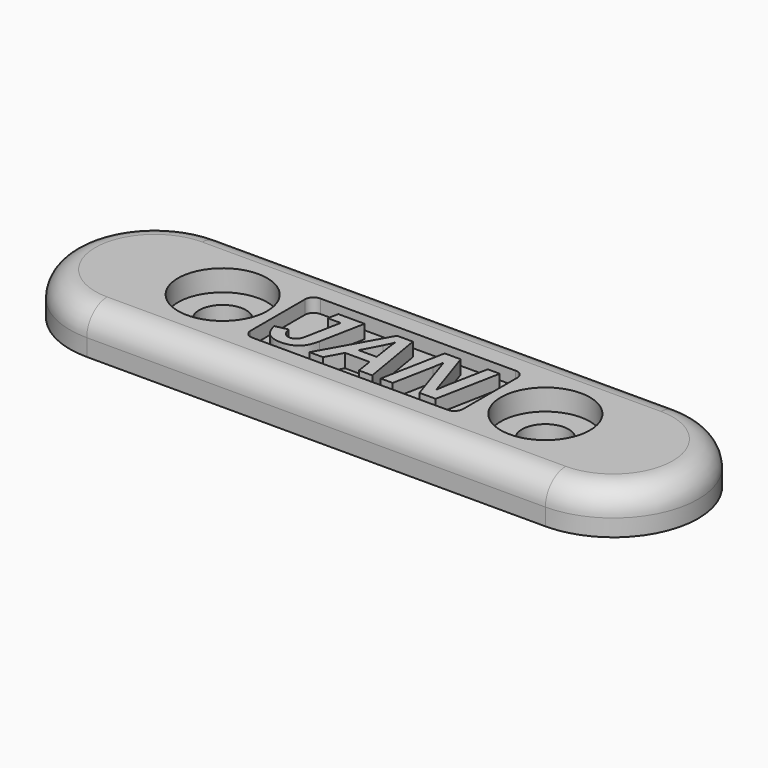
from build123d import *

# Parameters (mm, degrees)
F0_R     = 5.25
F0_R_2   = 2.75
F1_DEPTH = 5
F2_DEPTH = 2.5
F4_R     = 3
F6_DEPTH = 1.6


with BuildPart() as f1:
    # F0 (on Top) → F1 (new body)
    with BuildSketch(Plane.XY):
        with BuildLine():
            Line((27, 10), (-27, 10))
            ThreePointArc((-27, 10), (-37, 0), (-27, -10))
            Line((-27, -10), (27, -10))
            ThreePointArc((27, -10), (37, 0), (27, 10))
        make_face()
        with Locations((-19, 0)):
            Circle(F0_R, mode=Mode.SUBTRACT)
        with Locations((19, 0)):
            Circle(F0_R, mode=Mode.SUBTRACT)
        with Locations((-19, 0)):
            Circle(F0_R)
        with Locations((-19, 0)):
            Circle(F0_R_2, mode=Mode.SUBTRACT)
        with Locations((19, 0)):
            Circle(F0_R)
        with Locations((19, 0)):
            Circle(F0_R_2, mode=Mode.SUBTRACT)
    extrude(amount=-F1_DEPTH)

    # F0 (on Top) → F2 (cut)
    with BuildSketch(Plane.XY):
        with Locations((-19, 0)):
            Circle(F0_R)
        with Locations((-19, 0)):
            Circle(F0_R_2, mode=Mode.SUBTRACT)
        with Locations((19, 0)):
            Circle(F0_R)
        with Locations((19, 0)):
            Circle(F0_R_2, mode=Mode.SUBTRACT)
    extrude(amount=-F2_DEPTH, mode=Mode.SUBTRACT)

    # F4
    f4_edges = [f1.edges().sort_by_distance(p)[0] for p in [
        (0, -10, 0),
        (0, 10, 0),
    ]]
    fillet(f4_edges, radius=F4_R)

    # F5 (on face) → F6 (cut)
    with BuildSketch(Plane.XY):
        with BuildLine():
            Line((11.5, 5), (-11.5, 5))
            ThreePointArc((-11.5, 5), (-12.2071067812, 4.7071067812), (-12.5, 4))
            Line((-12.5, 4), (-12.5, -4))
            ThreePointArc((-12.5, -4), (-12.2071067812, -4.7071067812), (-11.5, -5))
            Line((-11.5, -5), (11.5, -5))
            ThreePointArc((11.5, -5), (12.2071067812, -4.7071067812), (12.5, -4))
            Line((12.5, -4), (12.5, 4))
            ThreePointArc((12.5, 4), (12.2071067812, 4.7071067812), (11.5, 5))
        make_face()
        with BuildLine():
            add(Edge.make_bspline(
                [(-7.1087151842, -3.5052785265), (-7.754492363, -4.0761455526), (-8.9168912848, -4.0761455526)],
                knots=[0, 0, 0, 1, 1, 1], degree=2))
            add(Edge.make_bspline(
                [(-8.9168912848, -4.0761455526), (-9.939802336, -4.0761455526), (-10.5502770291, -3.5586627733)],
                knots=[0, 0, 0, 1, 1, 1], degree=2))
            add(Edge.make_bspline(
                [(-10.5502770291, -3.5586627733), (-11.1607517221, -3.041179994), (-11.3656783468, -1.928721174)],
                knots=[0, 0, 0, 1, 1, 1], degree=2))
            Line((-11.3656783468, -1.928721174), (-9.9277478287, -1.6153039832))
            add(Edge.make_bspline(
                [(-9.9277478287, -1.6153039832), (-9.6814914645, -2.8328092243), (-8.8152890087, -2.8328092243)],
                knots=[0, 0, 0, 1, 1, 1], degree=2))
            add(Edge.make_bspline(
                [(-8.8152890087, -2.8328092243), (-8.5242587601, -2.8328092243), (-8.325359389, -2.7036537886)],
                knots=[0, 0, 0, 1, 1, 1], degree=2))
            add(Edge.make_bspline(
                [(-8.325359389, -2.7036537886), (-8.126460018, -2.5744983528), (-7.9973045822, -2.3377133872)],
                knots=[0, 0, 0, 1, 1, 1], degree=2))
            add(Edge.make_bspline(
                [(-7.9973045822, -2.3377133872), (-7.8681491465, -2.1009284217), (-7.7699910153, -1.5998053309)],
                knots=[0, 0, 0, 1, 1, 1], degree=2))
            Line((-7.7699910153, -1.5998053309), (-7.0002246181, 2.3712938005))
            Line((-7.0002246181, 2.3712938005), (-8.5139263252, 2.3712938005))
            Line((-8.5139263252, 2.3712938005), (-8.2762803235, 3.6146301288))
            Line((-8.2762803235, 3.6146301288), (-5.1817160827, 3.6146301288))
            Line((-5.1817160827, 3.6146301288), (-6.2201257862, -1.6910751722))
            add(Edge.make_bspline(
                [(-6.2201257862, -1.6910751722), (-6.4629380054, -2.9344115004), (-7.1087151842, -3.5052785265)],
                knots=[0, 0, 0, 1, 1, 1], degree=2))
        make_face(mode=Mode.SUBTRACT)
        Polygon((1.7909553759, -3.9676549865), (0.220425277, -3.9676549865), (-0.075771189, -2.0303234501), (-2.965408805, -2.0303234501), (-4.0141509434, -3.9676549865), (-5.5967355496, -3.9676549865), (-1.3621593291, 3.6146301288), (0.5114555256, 3.6146301288), align=None, mode=Mode.SUBTRACT)
        with BuildLine():
            Line((9.2613057802, -3.9676549865), (7.346361186, -3.9676549865))
            Line((7.346361186, -3.9676549865), (5.3332584606, 2.1181491465))
            add(Edge.make_bspline(
                [(5.3332584606, 2.1181491465), (5.2092692423, 1.2467804732), (5.1283318359, 0.8334830788)],
                knots=[0, 0, 0, 1, 1, 1], degree=2))
            Line((5.1283318359, 0.8334830788), (4.1915244085, -3.9676549865))
            Line((4.1915244085, -3.9676549865), (2.7828691225, -3.9676549865))
            Line((2.7828691225, -3.9676549865), (4.2569631626, 3.6146301288))
            Line((4.2569631626, 3.6146301288), (6.1409104522, 3.6146301288))
            Line((6.1409104522, 3.6146301288), (8.1695118299, -2.524558251))
            Line((8.1695118299, -2.524558251), (8.2332285115, -2.0837076969))
            add(Edge.make_bspline(
                [(8.2332285115, -2.0837076969), (8.2935010482, -1.6376909254), (8.3899371069, -1.1469002695)],
                knots=[0, 0, 0, 1, 1, 1], degree=2))
            Line((8.3899371069, -1.1469002695), (9.3267445343, 3.6146301288))
            Line((9.3267445343, 3.6146301288), (10.7353998203, 3.6146301288))
            Line((10.7353998203, 3.6146301288), (9.2613057802, -3.9676549865))
        make_face(mode=Mode.SUBTRACT)
        with BuildLine():
            add(Edge.make_bspline(
                [(-0.559673555, 1.596361186), (-0.6561096137, 2.3230757712), (-0.6561096137, 2.4470649895)],
                knots=[0, 0, 0, 1, 1, 1], degree=2))
            add(Edge.make_bspline(
                [(-0.6561096137, 2.4470649895), (-0.7697663971, 2.1026504942), (-1.184785864, 1.3070530099)],
                knots=[0, 0, 0, 1, 1, 1], degree=2))
            Line((-1.184785864, 1.3070530099), (-2.3247978437, -0.8352051512))
            Line((-2.3247978437, -0.8352051512), (-0.1997604073, -0.8352051512))
            Line((-0.1997604073, -0.8352051512), (-0.559673555, 1.596361186))
        make_face()
    extrude(amount=-F6_DEPTH, mode=Mode.SUBTRACT)


solid = f1.part
